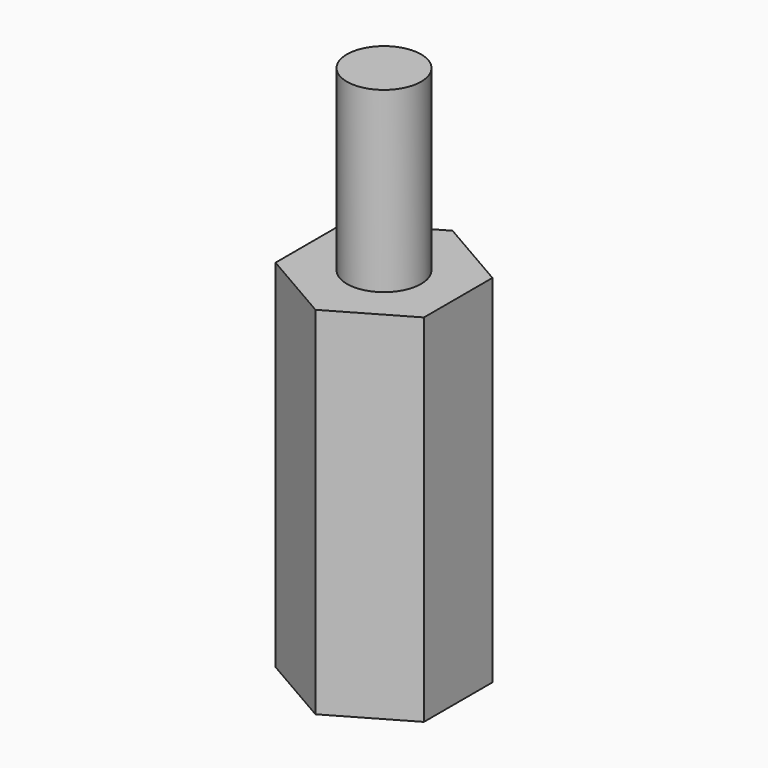
from build123d import *

# Parameters (mm, degrees)
F1_DEPTH = 12
F2_R     = 1.25
F3_DEPTH = 6
F5_D     = 2.5
F5_DEPTH = 5
F5_TIP   = 0.7510757738


with BuildPart() as f1:
    # F0 (on Top) → F1 (new body)
    with BuildSketch(Plane.XY):
        Polygon((2.5, 1.443375673), (0, 2.8867513459), (-2.5, 1.443375673), (-2.5, -1.443375673), (0, -2.8867513459), (2.5, -1.443375673), align=None)
    extrude(amount=F1_DEPTH)

    # F2 (on face) → F3 (join)
    with BuildSketch(Plane.XY.offset(12)):
        Circle(F2_R)
    extrude(amount=F3_DEPTH)

    # F5
    with Locations(Plane(origin=(0, 0, 0), x_dir=(1, 0, 0), z_dir=(0, 0, -1))):
        with Locations((0, 0)):
            Hole(F5_D / 2, depth=F5_DEPTH)
            with Locations((0, 0, -(F5_DEPTH + F5_TIP / 2))):  # 118° drill point
                Cone(0, F5_D / 2, F5_TIP, mode=Mode.SUBTRACT)


solid = f1.part
